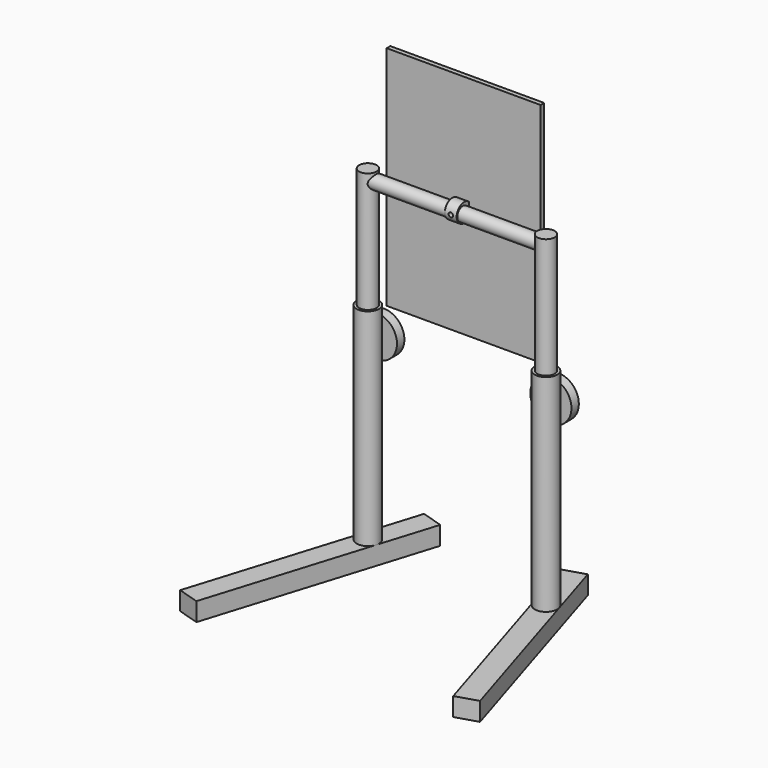
from build123d import *

# Parameters (mm, degrees)
F1_DEPTH  = 5.588
F2_R      = 3.400863531
F3_DEPTH  = 62.484
F4_R      = 2.6358793968
F5_DEPTH  = 36.322
F6_R      = 2.0902316786
F7_DEPTH  = 26.4668
F9_W      = 46.5320684016
F9_H      = 68.596586585
F10_DEPTH = 1.3716
F11_R     = 6.2245067114
F12_DEPTH = 2.794
F14_DEPTH = 1.778
F15_R     = 0.6779698322
F16_DEPTH = 3.7084
F17_DEPTH = 6.1214


with BuildPart() as f1:
    # F0 (on Top) → F1 (new body)
    with BuildSketch(Plane.XY):
        Polygon((24.754703592, 18.5309260663), (18.2574551058, 16.5186504552), (38.8415608429, -49.9434430581), (45.338809329, -47.931167447), align=None)
    extrude(amount=F1_DEPTH)

    # F2 (on face) → F3 (join)
    with BuildSketch(Plane.XY.offset(5.588)):
        with Locations((26.9337159988, 0)):
            Circle(F2_R)
    extrude(amount=F3_DEPTH)


with BuildPart() as f1b:
    # F0 (on Top) → F1, piece 2 (new body)
    with BuildSketch(Plane.XY):
        Polygon((-24.754703592, 18.5309260663), (-45.338809329, -47.931167447), (-38.8415608429, -49.9434430581), (-18.2574551058, 16.5186504552), align=None)
    extrude(amount=F1_DEPTH)


with BuildPart() as f3:
    # F2 (on face) → F3, piece 2 (new body)
    with BuildSketch(Plane.XY.offset(5.588)):
        with Locations((-26.9337159988, 0)):
            Circle(F2_R)
    extrude(amount=F3_DEPTH)


with BuildPart() as f5:
    # F4 (on face) → F5 (new body)
    with BuildSketch(Plane.XY.offset(68.072)):
        with Locations((26.9337159988, 0)):
            Circle(F4_R)
    extrude(amount=F5_DEPTH)


with BuildPart() as f5b:
    # F4 (on face) → F5, piece 2 (new body)
    with BuildSketch(Plane.XY.offset(68.072)):
        with Locations((-26.9337159988, 0)):
            Circle(F4_R)
    extrude(amount=F5_DEPTH)


with BuildPart() as f7:
    # F6 (on Right) → F7 (new body, symmetric)
    with BuildSketch(Plane.YZ):
        with Locations((0, 101.6435548663)):
            Circle(F6_R)
    extrude(amount=F7_DEPTH, both=True)

    # F13 (on Right) → F14 (join, symmetric)
    with BuildSketch(Plane.YZ):
        with BuildLine():
            Line((2.3708415683, 99.6423438191), (2.4390823673, 103.782273829))
            ThreePointArc((2.4390823673, 103.782273829), (-2.3216692714, 101.79022055), (2.3708415683, 99.6423438191))
        make_face()
    extrude(amount=F14_DEPTH, both=True)

    # F15 (on Front) → F16 (cut)
    with BuildSketch(Plane.XZ):
        with Locations((0, 101.6723290086)):
            Circle(F15_R)
    extrude(amount=F16_DEPTH, mode=Mode.SUBTRACT)

    # F17 (cut): a face of the model
    f17_faces = [f7.faces().sort_by_distance(p)[0] for p in [
        (0, 0, 101.6723290086),
    ]]
    extrude(f17_faces, amount=-F17_DEPTH, mode=Mode.SUBTRACT)


with BuildPart() as f10:
    # F9 (on offset) → F10 (new body)
    with BuildSketch(Plane.XZ.offset(-2.54)):
        with Locations((0, 102.2457927465)):
            Rectangle(F9_W, F9_H)
    extrude(amount=-F10_DEPTH)


with BuildPart() as f12:
    # F11 (on offset) → F12 (new body)
    with BuildSketch(Plane.XZ.offset(-2.54)):
        with Locations((26.3785496354, 58.8667541742)):
            Circle(F11_R)
    extrude(amount=-F12_DEPTH)


with BuildPart() as f12b:
    # F11 (on offset) → F12, piece 2 (new body)
    with BuildSketch(Plane.XZ.offset(-2.54)):
        with Locations((-26.3785496354, 58.8667541742)):
            Circle(F11_R)
    extrude(amount=-F12_DEPTH)


solid = Compound([f1.part, f1b.part, f3.part, f5.part, f5b.part, f7.part, f10.part, f12.part, f12b.part])
